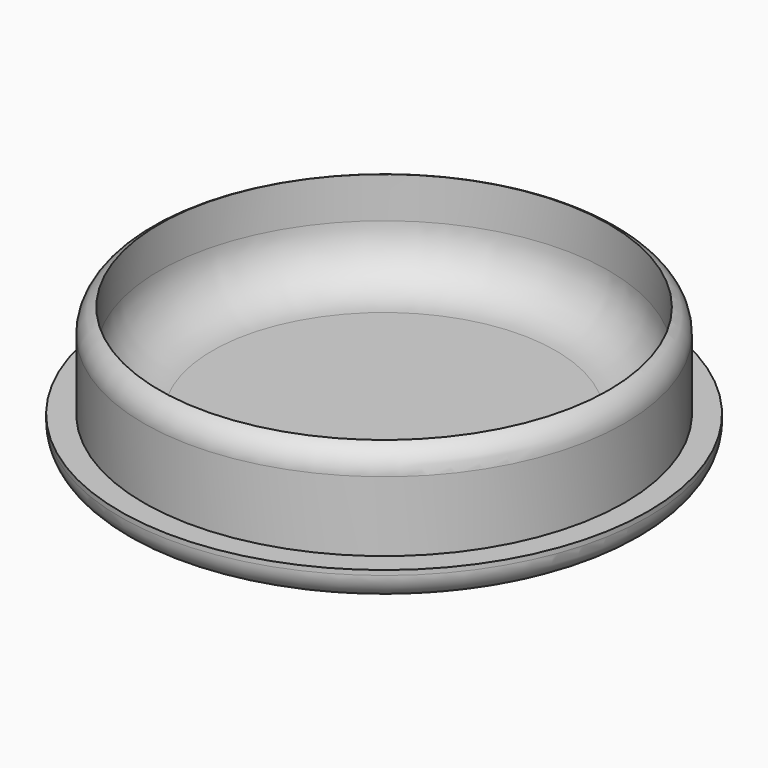
from build123d import *

# Parameters (mm, degrees)
F0_R     = 25.25
F1_DEPTH = 3
F2_R     = 23
F2_R_2   = 21.5
F3_DEPTH = 9
F4_R     = 2.54
F6_R     = 5.08


# Not quite as in the source:
# - a fillet or chamfer that OpenCascade refuses, or shapes differently, is made with other operations: its cross-section is extruded or revolved along the edge and cut away or added


with BuildPart() as f1:
    # F0 (on Top) → F1 (new body)
    with BuildSketch(Plane.XY):
        Circle(F0_R)
    extrude(amount=F1_DEPTH)

    # F2 (on face) → F3 (join)
    with BuildSketch(Plane.XY.offset(3)):
        Circle(F2_R)
        Circle(F2_R_2, mode=Mode.SUBTRACT)
    extrude(amount=F3_DEPTH)

    # F4
    f4_edges = [f1.edges().sort_by_distance(p)[0] for p in [
        (-25.25, 0, 0),
    ]]
    fillet(f4_edges, radius=F4_R)

    # F5: fillet of radius 2.54 on 1 edges, made by hand

    # F5_s1 → F5_t2 (revolve, cut)
    with BuildSketch(Plane.XZ):
        with BuildLine():
            ThreePointArc((23, 9.6826739547), (22.5922757795, 11.0628913289), (21.5, 12))
            Line((21.5, 12), (23, 12))
            Line((23, 12), (23, 9.6826739547))
        make_face()
    revolve(axis=Axis((0, 0, 12), (0, 0, 1)), mode=Mode.SUBTRACT)

    # F6
    f6_edges = [f1.edges().sort_by_distance(p)[0] for p in [
        (-21.5, 0, 3),
    ]]
    fillet(f6_edges, radius=F6_R)


solid = f1.part
